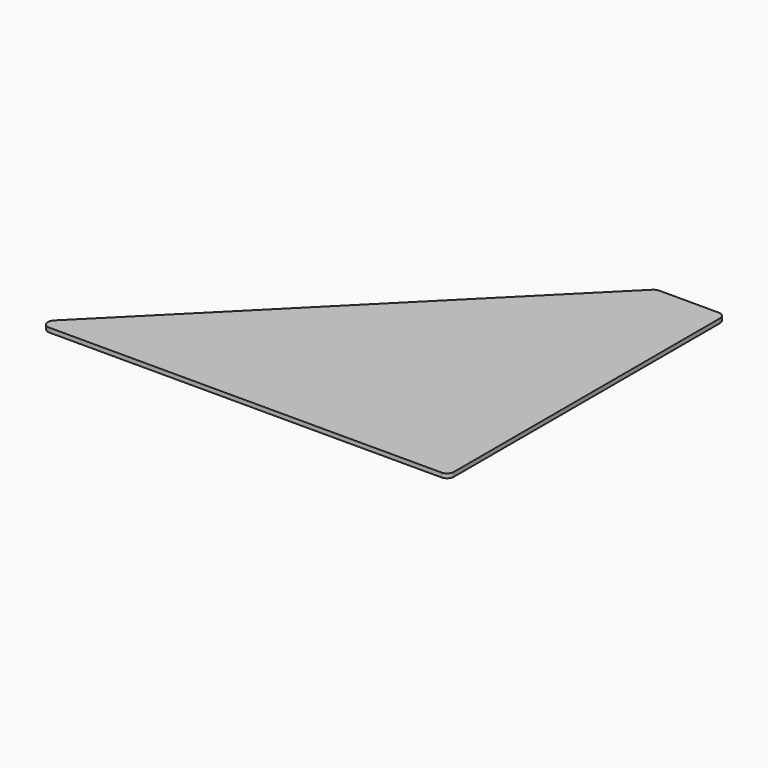
from build123d import *

# Parameters (mm, degrees)
F1_DEPTH = 3.175
F2_R     = 5.08


# Not quite as in the source:
# - a length typed as a fraction of an inch, garbled in the dataset ("3 / 203.2 mm" for 3/8 in), is restored


with BuildPart() as f1:
    # F0 (on Top) → F1 (new body)
    with BuildSketch(Plane.XY):
        Polygon((137.6824020138, -22.0465916001), (137.6824020138, 231.9534083999), (86.8824020138, 231.9534083999), (-167.1175979862, -22.0465916001), align=None)
    extrude(amount=F1_DEPTH)

    # F2
    f2_edges = [f1.edges().sort_by_distance(p)[0] for p in [
        (86.882402, 231.953408, 1.5875),
        (137.682402, 231.953408, 1.5875),
        (137.682402, -22.046592, 1.5875),
        (-167.117598, -22.046592, 1.5875),
    ]]
    fillet(f2_edges, radius=F2_R)


solid = f1.part
